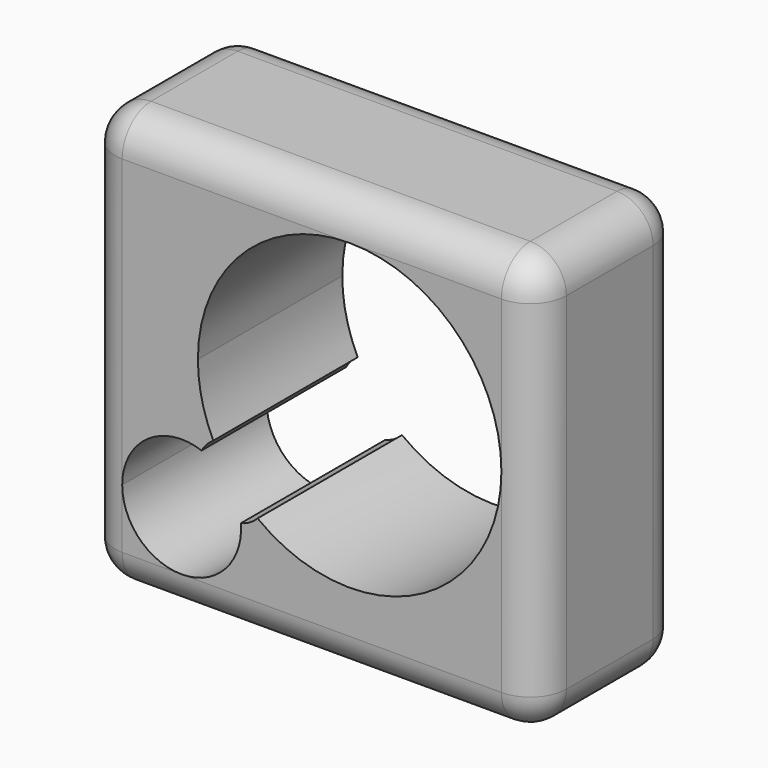
from build123d import *

# Parameters (mm, degrees)
F0_W         = 63.5255295783
F0_H         = 58.9018370956
F1_DEPTH     = 25.4
F2_R         = 5.08
F3_R         = 5.08
F4_T1_DEPTH  = 15.24
F4_S5_W      = 5.08
F4_S5_H      = 5.08
F4_T6_DEPTH  = 5.08
F4_S11_W     = 5.08
F4_S11_H     = 5.08
F4_T12_DEPTH = 5.08
F4_S17_W     = 5.08
F4_S17_H     = 5.08
F4_T18_DEPTH = 5.08
F4_S23_W     = 5.08
F4_S23_H     = 5.08
F4_T24_DEPTH = 5.08
F4_S29_W     = 5.08
F4_S29_H     = 5.08
F4_T30_DEPTH = 5.08
F4_S35_W     = 5.08
F4_S35_H     = 5.08
F4_T36_DEPTH = 5.08
F4_S41_W     = 5.08
F4_S41_H     = 5.08
F4_T42_DEPTH = 5.08
F4_S47_W     = 5.08
F4_S47_H     = 5.08
F4_T48_DEPTH = 5.08
F6_DEPTH     = 25.401


# Not quite as in the source:
# - a fillet or chamfer that OpenCascade refuses, or shapes differently, is made with other operations: its cross-section is extruded or revolved along the edge and cut away or added


with BuildPart() as f1:
    # F0 (on Front) → F1 (new body)
    with BuildSketch(Plane.XZ):
        with Locations((7.1365712211, -3.0154520646)):
            Rectangle(F0_W, F0_H)
    extrude(amount=F1_DEPTH)

    # F2
    f2_edges = [f1.edges().sort_by_distance(p)[0] for p in [
        (7.136571, -25.4, 26.435466),
        (-24.626194, -25.4, -3.015452),
        (7.136571, -25.4, -32.466371),
        (38.899336, -25.4, -3.015452),
    ]]
    fillet(f2_edges, radius=F2_R)

    # F3
    f3_edges = [f1.edges().sort_by_distance(p)[0] for p in [
        (7.136571, 0, 26.435466),
        (38.899336, 0, -3.015452),
        (-24.626194, 0, -3.015452),
        (7.136571, 0, -32.466371),
    ]]
    fillet(f3_edges, radius=F3_R)

    # F4: fillet of radius 5.08 on 4 edges, made by hand

    # F4_s2 → F4_t1 (cut)
    with BuildSketch(Plane.XZ.offset(5.08)):
        with BuildLine():
            ThreePointArc((33.8193360102, 26.4354664832), (37.4114384586, 24.9475689317), (38.8993360102, 21.3554664832))
            Line((38.8993360102, 21.3554664832), (38.8993360102, 26.4354664832))
            Line((38.8993360102, 26.4354664832), (33.8193360102, 26.4354664832))
        make_face()
        with BuildLine():
            ThreePointArc((38.8993360102, -27.3863706124), (37.4114384586, -30.9784730608), (33.8193360102, -32.4663706124))
            Line((33.8193360102, -32.4663706124), (38.8993360102, -32.4663706124))
            Line((38.8993360102, -32.4663706124), (38.8993360102, -27.3863706124))
        make_face()
        with BuildLine():
            ThreePointArc((-19.5461935681, 26.4354664832), (-23.1382960165, 24.9475689317), (-24.6261935681, 21.3554664832))
            Line((-24.6261935681, 21.3554664832), (-24.6261935681, 26.4354664832))
            Line((-24.6261935681, 26.4354664832), (-19.5461935681, 26.4354664832))
        make_face()
        with BuildLine():
            ThreePointArc((-24.6261935681, -27.3863706124), (-23.1382960165, -30.9784730608), (-19.5461935681, -32.4663706124))
            Line((-19.5461935681, -32.4663706124), (-24.6261935681, -32.4663706124))
            Line((-24.6261935681, -32.4663706124), (-24.6261935681, -27.3863706124))
        make_face()
    extrude(amount=F4_T1_DEPTH, mode=Mode.SUBTRACT)


with BuildPart() as f4_tool4:
    # F4_s5 → F4_t6 (new body)
    with BuildSketch(Plane.YZ.offset(-19.5461935681)):
        with Locations((-2.54, -29.9263706124)):
            Rectangle(F4_S5_W, F4_S5_H)
    extrude(amount=-F4_T6_DEPTH)

    # F4_s7 → F4_t8 (revolve, cut)
    with BuildSketch(Plane(origin=(-19.5461935681, -5.08, -27.3863706124), x_dir=(0, -0.7071067812, 0.7071067812), z_dir=(0, -0.7071067812, -0.7071067812))):
        with BuildLine():
            ThreePointArc((0, -5.08), (5.08, 0), (0, 5.08))
            Line((0, 5.08), (0, -5.08))
        make_face()
    revolve(axis=Axis((-19.5461935681, -5.08, -27.3863706124), (-1, 0, 0)), mode=Mode.SUBTRACT)


with BuildPart() as f1_1:
    add(f1.part)

    # F4_t3: cut F4_tool4
    add(f4_tool4.part, mode=Mode.SUBTRACT)


with BuildPart() as f4_tool10:
    # F4_s11 → F4_t12 (new body)
    with BuildSketch(Plane.YZ.offset(-19.5461935681)):
        with Locations((-22.86, -29.9263706124)):
            Rectangle(F4_S11_W, F4_S11_H)
    extrude(amount=-F4_T12_DEPTH)

    # F4_s13 → F4_t14 (revolve, cut)
    with BuildSketch(Plane(origin=(-19.5461935681, -20.32, -27.3863706124), x_dir=(0, 0.7071067812, 0.7071067812), z_dir=(0, -0.7071067812, 0.7071067812))):
        with BuildLine():
            ThreePointArc((0, -5.08), (5.08, 0), (0, 5.08))
            Line((0, 5.08), (0, -5.08))
        make_face()
    revolve(axis=Axis((-19.5461935681, -20.32, -27.3863706124), (-1, 0, 0)), mode=Mode.SUBTRACT)


with BuildPart() as f1_2:
    add(f1_1.part)

    # F4_t9: cut F4_tool10
    add(f4_tool10.part, mode=Mode.SUBTRACT)


with BuildPart() as f4_tool16:
    # F4_s17 → F4_t18 (new body)
    with BuildSketch(Plane.XY.offset(21.3554664832)):
        with Locations((-22.0861935681, -2.54)):
            Rectangle(F4_S17_W, F4_S17_H)
    extrude(amount=F4_T18_DEPTH)

    # F4_s19 → F4_t20 (revolve, cut)
    with BuildSketch(Plane(origin=(-19.5461935681, -5.08, 21.3554664832), x_dir=(0.7071067812, -0.7071067812, 0), z_dir=(-0.7071067812, -0.7071067812, 0))):
        with BuildLine():
            ThreePointArc((0, -5.08), (5.08, 0), (0, 5.08))
            Line((0, 5.08), (0, -5.08))
        make_face()
    revolve(axis=Axis((-19.5461935681, -5.08, 21.3554664832), (0, 0, 1)), mode=Mode.SUBTRACT)


with BuildPart() as f1_3:
    add(f1_2.part)

    # F4_t15: cut F4_tool16
    add(f4_tool16.part, mode=Mode.SUBTRACT)


with BuildPart() as f4_tool22:
    # F4_s23 → F4_t24 (new body)
    with BuildSketch(Plane.XY.offset(21.3554664832)):
        with Locations((-22.0861935681, -22.86)):
            Rectangle(F4_S23_W, F4_S23_H)
    extrude(amount=F4_T24_DEPTH)

    # F4_s25 → F4_t26 (revolve, cut)
    with BuildSketch(Plane(origin=(-19.5461935681, -20.32, 21.3554664832), x_dir=(0.7071067812, 0.7071067812, 0), z_dir=(0.7071067812, -0.7071067812, 0))):
        with BuildLine():
            ThreePointArc((0, -5.08), (5.08, 0), (0, 5.08))
            Line((0, 5.08), (0, -5.08))
        make_face()
    revolve(axis=Axis((-19.5461935681, -20.32, 21.3554664832), (0, 0, 1)), mode=Mode.SUBTRACT)


with BuildPart() as f1_4:
    add(f1_3.part)

    # F4_t21: cut F4_tool22
    add(f4_tool22.part, mode=Mode.SUBTRACT)


with BuildPart() as f4_tool28:
    # F4_s29 → F4_t30 (new body)
    with BuildSketch(Plane.YZ.offset(33.8193360102)):
        with Locations((-2.54, -29.9263706124)):
            Rectangle(F4_S29_W, F4_S29_H)
    extrude(amount=F4_T30_DEPTH)

    # F4_s31 → F4_t32 (revolve, cut)
    with BuildSketch(Plane(origin=(33.8193360102, -5.08, -27.3863706124), x_dir=(0, -0.7071067812, 0.7071067812), z_dir=(0, 0.7071067812, 0.7071067812))):
        with BuildLine():
            ThreePointArc((0, -5.08), (5.08, 0), (0, 5.08))
            Line((0, 5.08), (0, -5.08))
        make_face()
    revolve(axis=Axis((33.8193360102, -5.08, -27.3863706124), (1, 0, 0)), mode=Mode.SUBTRACT)


with BuildPart() as f1_5:
    add(f1_4.part)

    # F4_t27: cut F4_tool28
    add(f4_tool28.part, mode=Mode.SUBTRACT)


with BuildPart() as f4_tool34:
    # F4_s35 → F4_t36 (new body)
    with BuildSketch(Plane.YZ.offset(33.8193360102)):
        with Locations((-22.86, -29.9263706124)):
            Rectangle(F4_S35_W, F4_S35_H)
    extrude(amount=F4_T36_DEPTH)

    # F4_s37 → F4_t38 (revolve, cut)
    with BuildSketch(Plane(origin=(33.8193360102, -20.32, -27.3863706124), x_dir=(0, 0.7071067812, 0.7071067812), z_dir=(0, 0.7071067812, -0.7071067812))):
        with BuildLine():
            ThreePointArc((0, -5.08), (5.08, 0), (0, 5.08))
            Line((0, 5.08), (0, -5.08))
        make_face()
    revolve(axis=Axis((33.8193360102, -20.32, -27.3863706124), (1, 0, 0)), mode=Mode.SUBTRACT)


with BuildPart() as f1_6:
    add(f1_5.part)

    # F4_t33: cut F4_tool34
    add(f4_tool34.part, mode=Mode.SUBTRACT)


with BuildPart() as f4_tool40:
    # F4_s41 → F4_t42 (new body)
    with BuildSketch(Plane.XY.offset(21.3554664832)):
        with Locations((36.3593360102, -2.54)):
            Rectangle(F4_S41_W, F4_S41_H)
    extrude(amount=F4_T42_DEPTH)

    # F4_s43 → F4_t44 (revolve, cut)
    with BuildSketch(Plane(origin=(33.8193360102, -5.08, 21.3554664832), x_dir=(-0.7071067812, -0.7071067812, 0), z_dir=(-0.7071067812, 0.7071067812, 0))):
        with BuildLine():
            ThreePointArc((0, -5.08), (5.08, 0), (0, 5.08))
            Line((0, 5.08), (0, -5.08))
        make_face()
    revolve(axis=Axis((33.8193360102, -5.08, 21.3554664832), (0, 0, 1)), mode=Mode.SUBTRACT)


with BuildPart() as f1_7:
    add(f1_6.part)

    # F4_t39: cut F4_tool40
    add(f4_tool40.part, mode=Mode.SUBTRACT)


with BuildPart() as f4_tool46:
    # F4_s47 → F4_t48 (new body)
    with BuildSketch(Plane.XY.offset(21.3554664832)):
        with Locations((36.3593360102, -22.86)):
            Rectangle(F4_S47_W, F4_S47_H)
    extrude(amount=F4_T48_DEPTH)

    # F4_s49 → F4_t50 (revolve, cut)
    with BuildSketch(Plane(origin=(33.8193360102, -20.32, 21.3554664832), x_dir=(-0.7071067812, 0.7071067812, 0), z_dir=(0.7071067812, 0.7071067812, 0))):
        with BuildLine():
            ThreePointArc((0, -5.08), (5.08, 0), (0, 5.08))
            Line((0, 5.08), (0, -5.08))
        make_face()
    revolve(axis=Axis((33.8193360102, -20.32, 21.3554664832), (0, 0, 1)), mode=Mode.SUBTRACT)


with BuildPart() as f1_8:
    add(f1_7.part)

    # F4_t45: cut F4_tool46
    add(f4_tool46.part, mode=Mode.SUBTRACT)

    # F5 (on face) → F6 (cut, through all)
    with BuildSketch(Plane(origin=(0, 0, 0), x_dir=(-1, 0, 0), z_dir=(0, 1, 0))):
        with BuildLine():
            ThreePointArc((6.7243616166, -9.373779083), (8.3427349026, -4.8105260449), (8.8915969563, 0))
            ThreePointArc((8.8915969563, 0), (-31.6040146397, 9.4715782097), (0.4899266998, -16.978077395))
            ThreePointArc((0.4899266998, -16.978077395), (0.2228411144, -10.4012847151), (6.7243616166, -9.373779083))
        make_face()
        with BuildLine():
            ThreePointArc((6.7243616166, -9.373779083), (0.2228411144, -10.4012847151), (0.4899266998, -16.978077395))
            ThreePointArc((0.4899266998, -16.978077395), (4.0507851492, -13.5396502777), (6.7243616166, -9.373779083))
        make_face()
        with BuildLine():
            ThreePointArc((6.7243616166, -9.373779083), (4.0507851492, -13.5396502777), (0.4899266998, -16.978077395))
            ThreePointArc((0.4899266998, -16.978077395), (1.5703386286, -17.823326152), (2.8412431673, -18.3395984162))
            ThreePointArc((2.8412431673, -18.3395984162), (4.5469228112, -13.9210498797), (8.3783969439, -11.136679181))
            ThreePointArc((8.3783969439, -11.136679181), (7.6606485066, -10.152707633), (6.7243616166, -9.373779083))
        make_face()
        with BuildLine():
            ThreePointArc((9.0007845368, -13.5396502777), (7.0934206735, -17.4441173353), (2.8412431673, -18.3395984162))
            ThreePointArc((2.8412431673, -18.3395984162), (10.8393587072, -27.3794387001), (19.5461935681, -19.0200373308))
            ThreePointArc((19.5461935681, -19.0200373308), (16.0046689137, -12.1850717648), (8.3783969439, -11.136679181))
            ThreePointArc((8.3783969439, -11.136679181), (8.842662113, -12.2985180922), (9.0007845368, -13.5396502777))
        make_face()
        with BuildLine():
            ThreePointArc((8.3783969439, -11.136679181), (4.5469228112, -13.9210498797), (2.8412431673, -18.3395984162))
            ThreePointArc((2.8412431673, -18.3395984162), (7.0934206735, -17.4441173353), (9.0007845368, -13.5396502777))
            ThreePointArc((9.0007845368, -13.5396502777), (8.842662113, -12.2985180922), (8.3783969439, -11.136679181))
        make_face()
    extrude(amount=-F6_DEPTH, mode=Mode.SUBTRACT)


solid = f1_8.part
